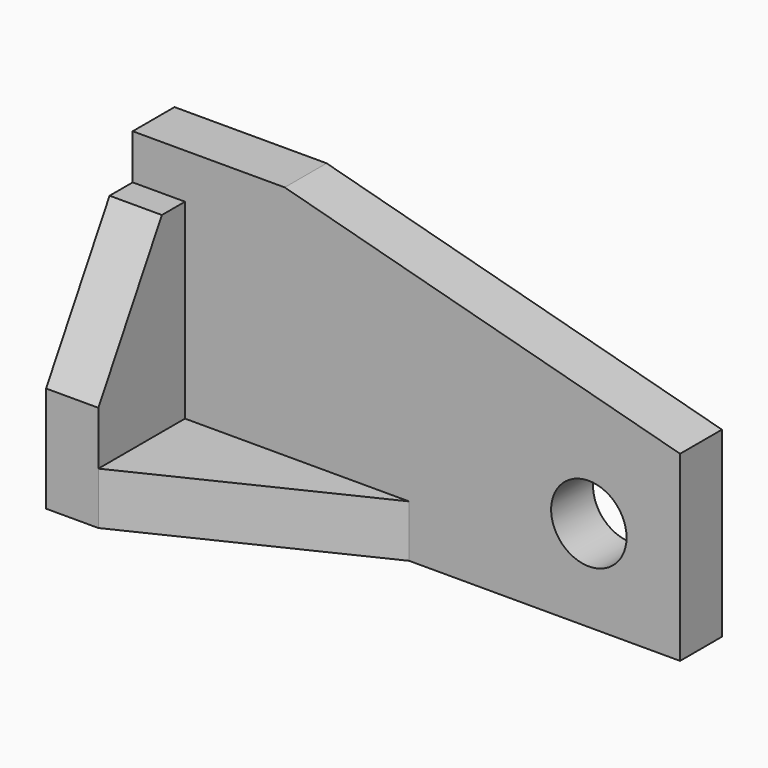
from build123d import *

# Parameters (mm, degrees)
F0_R        = 7.874
F1_DEPTH    = 10.922
F2_DEPTH    = 33.528
F0_W        = 10.922
F0_H        = 19.3979742137
F3_DEPTH    = 33.528
F4_SIZE2    = 16.5711074263
F4_SIZE     = 28.702
F5_T4_DEPTH = 283.3190140635


# Not quite as in the source:
# - a fillet or chamfer that OpenCascade refuses, or shapes differently, is made with other operations: its cross-section is extruded or revolved along the edge and cut away or added


with BuildPart() as f1:
    # F0 (on Front) → F1 (new body)
    with BuildSketch(Plane.XZ):
        Polygon((-43.8717590123, 47.7630699762), (-75.6217590123, 47.7630699762), (-75.6217590123, 38.3650699762), (-64.6997590123, 38.3650699762), (-64.6997590123, 18.9670957625), (-64.6997590123, -1.5129300238), (-12.1217590123, -1.5129300238), (-12.1217590123, -12.4349300238), (38.6782409877, -12.4349300238), (38.6782409877, 25.643864141), align=None)
        with Locations((19.6282409877, 6.6150699762)):
            Circle(F0_R, mode=Mode.SUBTRACT)
    extrude(amount=F1_DEPTH)

    # F0 (on Front) → F2 (join)
    with BuildSketch(Plane.XZ):
        Polygon((-43.8717590123, -12.4349300238), (-12.1217590123, -12.4349300238), (-12.1217590123, -1.5129300238), (-64.6997590123, -1.5129300238), (-64.6997590123, -12.4349300238), align=None)
    extrude(amount=F2_DEPTH)

    # F0 (on Front) → F3 (join)
    with BuildSketch(Plane.XZ):
        with Locations((-70.1607590123, 28.6660828693)):
            Rectangle(F0_W, F0_H)
        Polygon((-64.6997590123, 18.9670957625), (-75.6217590123, 18.9670957625), (-75.6217590123, -12.4349300238), (-64.6997590123, -12.4349300238), (-64.6997590123, -1.5129300238), align=None)
    extrude(amount=F3_DEPTH)

    # F4
    f4_edges = [f1.edges().sort_by_distance(p)[0] for p in [
        (-70.160759, -33.528, 38.36507),
    ]]
    f4_side = f1.faces().sort_by_distance((-70.160759, -33.528, 37.551873))[0]
    chamfer(f4_edges, length=F4_SIZE, length2=F4_SIZE2, reference=f4_side)

    # F5: chamfer of 25.4 x 52.578 on 1 edges, made by hand


with BuildPart() as f5_tool2:
    # F5_s3 → F5_t4 (new body)
    with BuildSketch(Plane.XY.offset(-148.6334370556)):
        Polygon((-64.6997590123, -33.528), (-12.1217590123, -8.128), (-12.1217590123, -33.528), align=None)
    extrude(amount=F5_T4_DEPTH)

    split(bisect_by=Plane.XZ.offset(10.922), keep=Keep.TOP)


with BuildPart() as f1_1:
    add(f1.part)

    # F5_t1: cut F5_tool2
    add(f5_tool2.part, mode=Mode.SUBTRACT)


solid = f1_1.part
